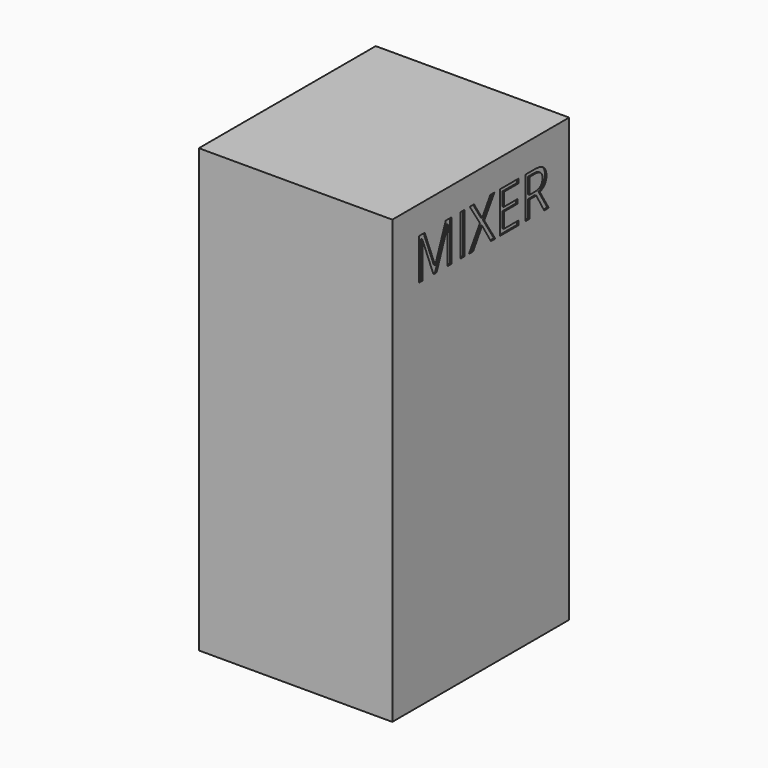
from build123d import *

# Parameters (mm, degrees)
F0_W         = 140
F0_H         = 160
F1_DEPTH     = 320
F3_TEXT_SIZE = 41.6666666667
F4_DEPTH     = 1


# Not quite as in the source:
# - Text() gives the source's letters only with a copy of the font that has no kerning and outlines rounded to 1/6400 em; it was checked with that copy


with BuildPart() as f1:
    # F0 (on Top) → F1 (new body)
    with BuildSketch(Plane.XY):
        Rectangle(F0_W, F0_H)
    extrude(amount=F1_DEPTH)

    # F3 (on face) → F4 (cut)
    with BuildSketch(Plane.YZ.offset(70)):
        with Locations((-60, 270)):
            Text('MIXER', F3_TEXT_SIZE, font='Open Sans', text_align=(TextAlign.LEFT, TextAlign.BOTTOM))
    extrude(amount=-F4_DEPTH, mode=Mode.SUBTRACT)


solid = f1.part
